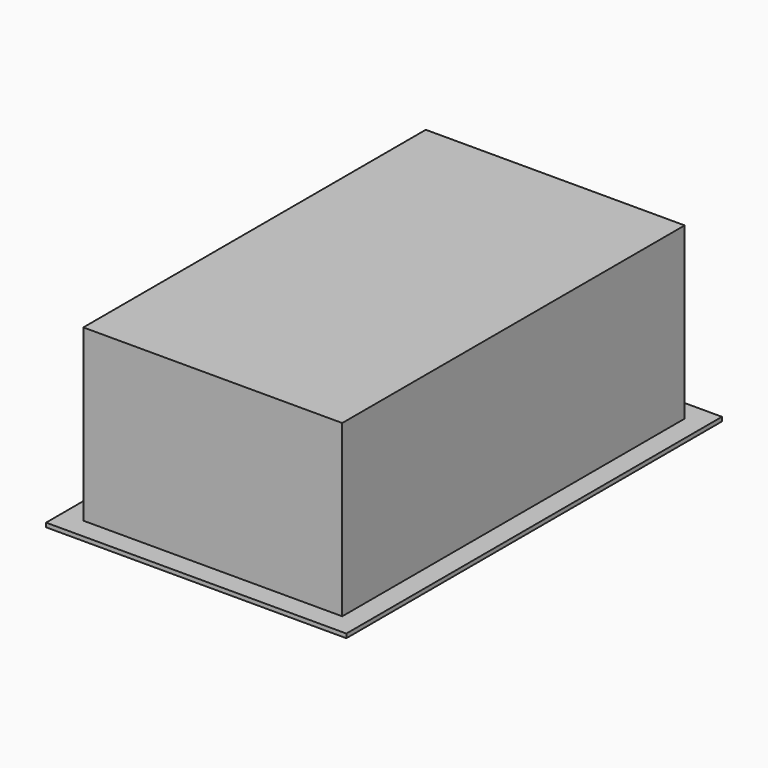
from build123d import *

# Parameters (mm, degrees)
F0_W        = 75
F0_H        = 124
F1_DEPTH    = 50.5
F0_W_2      = 87
F0_H_2      = 136
F2_DEPTH    = 1.2
F3_T        = 1.5
F3_T3_DEPTH = 78
F3_T5_DEPTH = 127


# Not quite as in the source:
# - a shell that OpenCascade refuses in one call is made with other operations: the cavity is built on its own and cut out


with BuildPart() as f1:
    # F0 (on Top) → F1 (new body)
    with BuildSketch(Plane.XY):
        with Locations((-11.4526251853, -17.2550516479)):
            Rectangle(F0_W, F0_H)
    extrude(amount=F1_DEPTH)

    # F0 (on Top) → F2 (join)
    with BuildSketch(Plane.XY):
        with Locations((-11.4526251853, -17.2550516479)):
            Rectangle(F0_W_2, F0_H_2)
        with Locations((-11.4526251853, -17.2550516479)):
            Rectangle(F0_W, F0_H, mode=Mode.SUBTRACT)
    extrude(amount=F2_DEPTH)

    # F3: shell of thickness 1.5, made by hand


with BuildPart() as f3_core1:
    # F3_t2: copy of F1
    add(f1.part)

    # the walls: a layer under each face that stays
    f3_faces = [f3_core1.faces().sort_by_distance(p)[0] for p in [
        (-11.4526251853, 44.7449483521, 25.85),
        (-52.0526251853, -80.7217183146, 1.2),
        (-48.9526251853, -17.2550516479, 25.85),
        (-11.4526251853, -17.2550516479, 50.5),
        (26.0473748147, -17.2550516479, 25.85),
        (-11.4526251853, -85.2550516479, 0.6),
        (32.0473748147, -17.2550516479, 0.6),
        (-11.4526251853, 50.7449483521, 0.6),
        (-54.9526251853, -17.2550516479, 0.6),
        (-11.4526251853, -79.2550516479, 25.85),
    ]]
    thicken(f3_faces, amount=-F3_T, mode=Mode.SUBTRACT)

    # F3_s4 → F3_t3 (cut)
    with BuildSketch(Plane.YZ.offset(-50.4526251853)):
        Polygon((44.7599483521, 1.215), (43.2449483521, 1.2), (43.2449483521, -0.3), (44.7449483521, -0.3), align=None)
        Polygon((-79.2700516479, 1.215), (-79.2550516479, -0.3), (-77.7550516479, -0.3), (-77.7550516479, 1.2), align=None)
    extrude(amount=F3_T3_DEPTH, mode=Mode.SUBTRACT)

    # F3_s6 → F3_t5 (cut)
    with BuildSketch(Plane.XZ.offset(-46.2449483521)):
        Polygon((26.0623748147, 1.215), (26.0473748147, -0.3), (24.5473748147, -0.3), (24.5473748147, 1.2), align=None)
        Polygon((-48.9676251853, 1.215), (-48.9526251853, -0.3), (-47.4526251853, -0.3), (-47.4526251853, 1.2), align=None)
    extrude(amount=F3_T5_DEPTH, mode=Mode.SUBTRACT)


with BuildPart() as f1_1:
    add(f1.part)

    # what is left inside the walls is the cavity
    f3_cavity = [f3_core1.part.solids().sort_by_distance(p)[0] for p in [
        (-11.452625, -37.421718, 0.015),
    ]]
    add(f3_cavity, mode=Mode.SUBTRACT)


solid = f1_1.part
